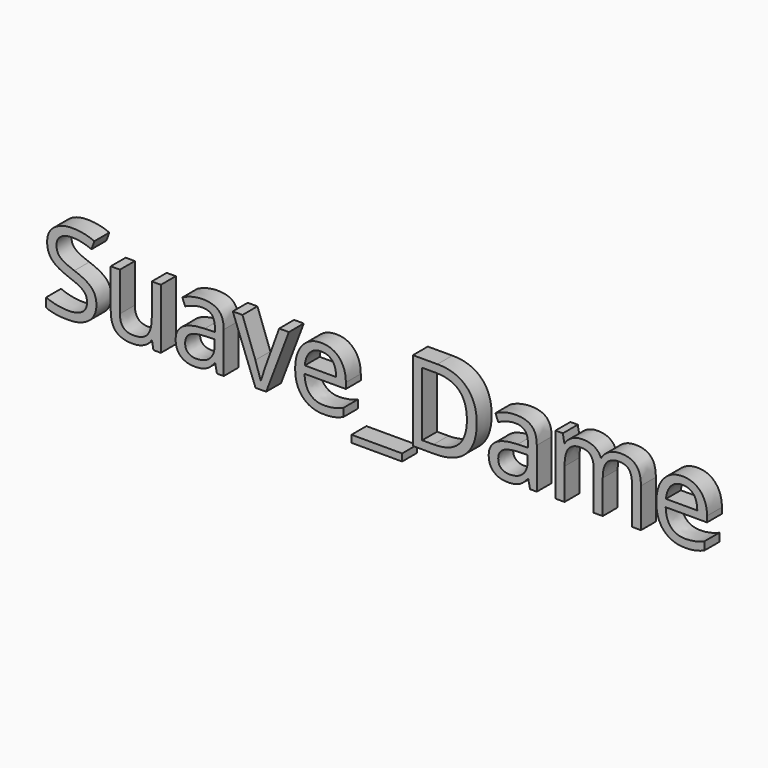
from build123d import *

# Parameters (mm, degrees)
F0_TEXT_SIZE = 15.2524521885
F1_DEPTH     = 2.54


# Not quite as in the source:
# - Text() gives the source's letters only with a copy of the font that has no kerning and outlines rounded to 1/6400 em; it was checked with that copy


with BuildPart() as f1:
    # F0 (on Front) → F1 (new body)
    with BuildSketch(Plane.XZ):
        with Locations((-34.2003516853, 7.216588594)):
            Text('Suave_Dame', F0_TEXT_SIZE, font='Open Sans', text_align=(TextAlign.LEFT, TextAlign.BOTTOM))
    extrude(amount=F1_DEPTH)


solid = f1.part
